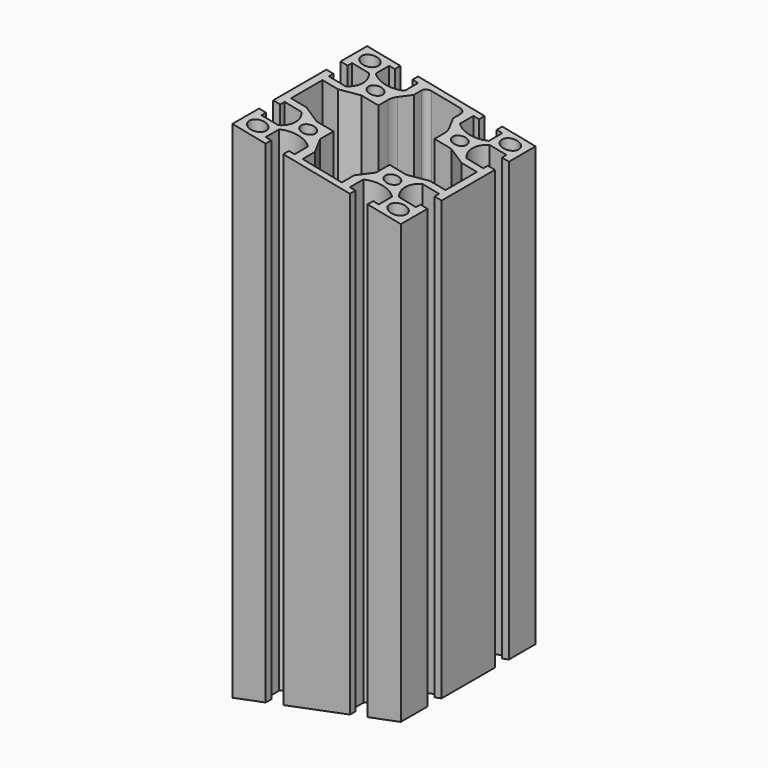
from build123d import *

# Parameters (mm, degrees)
F0_R          = 3
F0_R_2        = 2.5
F1_DEPTH      = 180
F2_R          = 2
F3_R          = 7
F6_DEPTH      = 30
F6_DEPTH_BACK = 30


# Not quite as in the source:
# - a feature names something its author has since deleted; it is built from what else it names


with BuildPart() as f1:
    # F0 (on Top) → F1 (new body)
    with BuildSketch(Plane.XY):
        with BuildLine():
            Line((18.15, -30), (30, -30))
            Line((30, -30), (30, -18.15))
            Line((30, -18.15), (27.5, -18.15))
            Line((27.5, -18.15), (27.5, -20.15))
            Line((27.5, -20.15), (21.5477069044, -20.15))
            ThreePointArc((21.5477069044, -20.15), (19.5, -15), (21.5477069044, -9.85))
            Line((21.5477069044, -9.85), (27.5, -9.85))
            Line((27.5, -9.85), (27.5, -11.85))
            Line((27.5, -11.85), (30, -11.85))
            Line((30, -11.85), (30, 11.85))
            Line((30, 11.85), (27.5, 11.85))
            Line((27.5, 11.85), (27.5, 9.85))
            Line((27.5, 9.85), (21.5477069044, 9.85))
            ThreePointArc((21.5477069044, 9.85), (19.5, 15), (21.5477069044, 20.15))
            Line((21.5477069044, 20.15), (27.5, 20.15))
            Line((27.5, 20.15), (27.5, 18.15))
            Line((27.5, 18.15), (30, 18.15))
            Line((30, 18.15), (30, 30))
            Line((30, 30), (18.15, 30))
            Line((18.15, 30), (18.15, 27.5))
            Line((18.15, 27.5), (20.15, 27.5))
            Line((20.15, 27.5), (20.15, 21.5477069044))
            ThreePointArc((20.15, 21.5477069044), (15, 19.5), (9.85, 21.5477069044))
            Line((9.85, 21.5477069044), (9.85, 27.5))
            Line((9.85, 27.5), (11.85, 27.5))
            Line((11.85, 27.5), (11.85, 30))
            Line((11.85, 30), (-11.85, 30))
            Line((-11.85, 30), (-11.85, 27.5))
            Line((-11.85, 27.5), (-9.85, 27.5))
            Line((-9.85, 27.5), (-9.85, 21.5477069044))
            ThreePointArc((-9.85, 21.5477069044), (-15, 19.5), (-20.15, 21.5477069044))
            Line((-20.15, 21.5477069044), (-20.15, 27.5))
            Line((-20.15, 27.5), (-18.15, 27.5))
            Line((-18.15, 27.5), (-18.15, 30))
            Line((-18.15, 30), (-30, 30))
            Line((-30, 30), (-30, 18.15))
            Line((-30, 18.15), (-27.5, 18.15))
            Line((-27.5, 18.15), (-27.5, 20.15))
            Line((-27.5, 20.15), (-21.5477069044, 20.15))
            ThreePointArc((-21.5477069044, 20.15), (-19.5, 15), (-21.5477069044, 9.85))
            Line((-21.5477069044, 9.85), (-27.5, 9.85))
            Line((-27.5, 9.85), (-27.5, 11.85))
            Line((-27.5, 11.85), (-30, 11.85))
            Line((-30, 11.85), (-30, -11.85))
            Line((-30, -11.85), (-27.5, -11.85))
            Line((-27.5, -11.85), (-27.5, -9.85))
            Line((-27.5, -9.85), (-21.5477069044, -9.85))
            ThreePointArc((-21.5477069044, -9.85), (-19.5, -15), (-21.5477069044, -20.15))
            Line((-21.5477069044, -20.15), (-27.5, -20.15))
            Line((-27.5, -20.15), (-27.5, -18.15))
            Line((-27.5, -18.15), (-30, -18.15))
            Line((-30, -18.15), (-30, -30))
            Line((-30, -30), (-18.15, -30))
            Line((-18.15, -30), (-18.15, -27.5))
            Line((-18.15, -27.5), (-20.15, -27.5))
            Line((-20.15, -27.5), (-20.15, -21.5477069044))
            ThreePointArc((-20.15, -21.5477069044), (-15, -19.5), (-9.85, -21.5477069044))
            Line((-9.85, -21.5477069044), (-9.85, -27.5))
            Line((-9.85, -27.5), (-11.85, -27.5))
            Line((-11.85, -27.5), (-11.85, -30))
            Line((-11.85, -30), (11.85, -30))
            Line((11.85, -30), (11.85, -27.5))
            Line((11.85, -27.5), (9.85, -27.5))
            Line((9.85, -27.5), (9.85, -21.5477069044))
            ThreePointArc((9.85, -21.5477069044), (15, -19.5), (20.15, -21.5477069044))
            Line((20.15, -21.5477069044), (20.15, -27.5))
            Line((20.15, -27.5), (18.15, -27.5))
            Line((18.15, -27.5), (18.15, -30))
        make_face()
        with Locations((-25, -25)):
            Circle(F0_R, mode=Mode.SUBTRACT)
        with Locations((-15, -15)):
            Circle(F0_R_2, mode=Mode.SUBTRACT)
        with Locations((25, -25)):
            Circle(F0_R, mode=Mode.SUBTRACT)
        with Locations((15, -15)):
            Circle(F0_R_2, mode=Mode.SUBTRACT)
        with Locations((-25, 25)):
            Circle(F0_R, mode=Mode.SUBTRACT)
        with Locations((-15, 15)):
            Circle(F0_R_2, mode=Mode.SUBTRACT)
        Polygon((-7, 22), (-7, 27.5), (0, 27.5), (7, 27.5), (7, 22), (10, 16), (10, 10), (16, 10), (22, 7), (27.5, 7), (27.5, 0), (27.5, -7), (22, -7), (16, -10), (10, -10), (10, -16), (7, -22), (7, -27.5), (0, -27.5), (-7, -27.5), (-7, -22), (-10, -16), (-10, -10), (-16, -10), (-22, -7), (-27.5, -7), (-27.5, 0), (-27.5, 7), (-22, 7), (-16, 10), (-10, 10), (-10, 16), align=None, mode=Mode.SUBTRACT)
        with Locations((15, 15)):
            Circle(F0_R_2, mode=Mode.SUBTRACT)
        with Locations((25, 25)):
            Circle(F0_R, mode=Mode.SUBTRACT)
    extrude(amount=F1_DEPTH)

    # F2
    f2_edges = [f1.edges().sort_by_distance(p)[0] for p in [
        (-7, 27.5, 90),
        (7, 27.5, 90),
    ]]
    fillet(f2_edges, radius=F2_R)

    # F3
    f3_edges = [f1.edges().sort_by_distance(p)[0] for p in [
        (-10, 16, 90),
        (10, 16, 90),
    ]]
    fillet(f3_edges, radius=F3_R)

    # F5 (on Front) → F6 (cut, two sides)
    with BuildSketch(Plane.XZ) as f6_sk:
        Polygon((79.680713533, 21.8168503847), (-30, 0), (-17.5886362159, -62.3961393031), (92.0920773171, -40.5792889183), align=None)
        Polygon((97.6667223127, 202.7474358776), (-20.7884412878, 226.3096328978), (-30, 180), (88.4551636005, 156.4378029799), align=None)
    extrude(amount=F6_DEPTH, mode=Mode.SUBTRACT)
    extrude(f6_sk.sketch, amount=-F6_DEPTH_BACK, mode=Mode.SUBTRACT)


solid = f1.part
